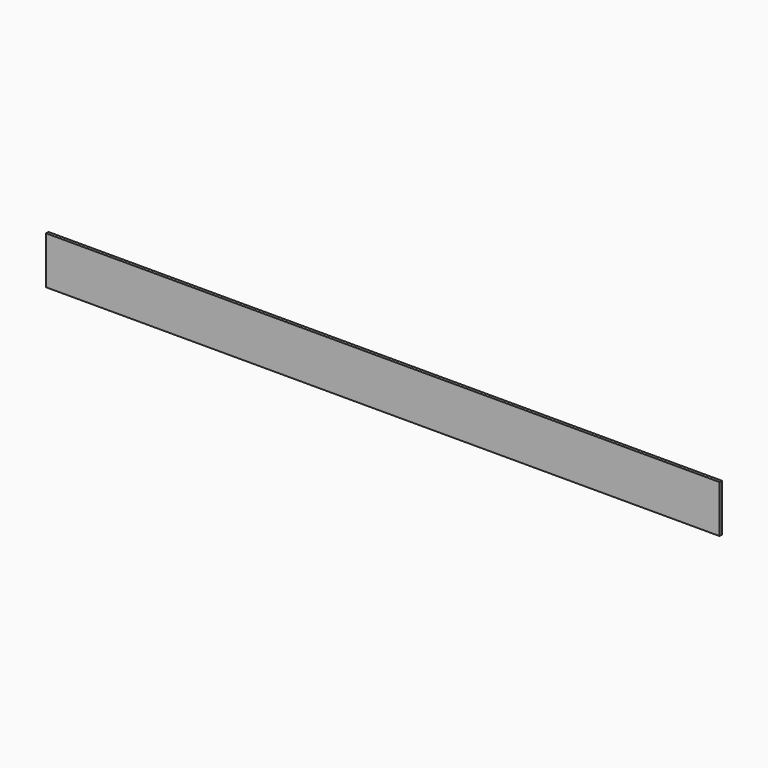
from build123d import *

# Parameters (mm, degrees)
F3_DEPTH = 340


# Not quite as in the source:
# - the program builds the solid bodies; features that only make, move or delete a surface that nothing else refers to are left out


with BuildPart() as f3:
    # F2 (on Right) → F3 (new body)
    with BuildSketch(Plane.YZ):
        Polygon((0, 12), (0, 0), (0, -12), (1.5, -12), (1.5, 12), align=None)
    extrude(amount=-F3_DEPTH)


solid = f3.part
